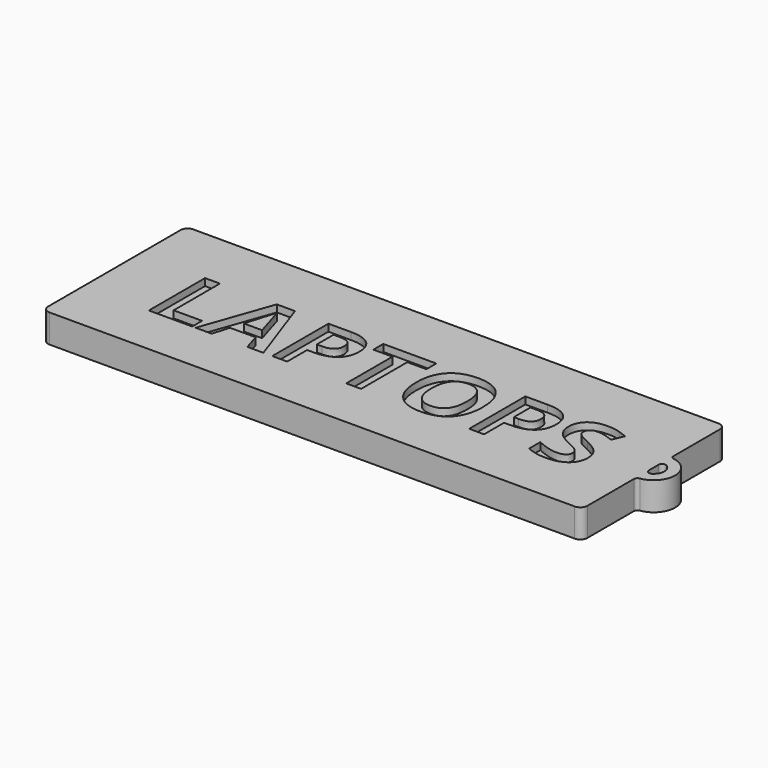
from build123d import *

# Parameters (mm, degrees)
F1_DEPTH     = 8
F2_TEXT_SIZE = 27.7777777778
F3_DEPTH     = 2


# Not quite as in the source:
# - Text() gives the source's letters only with a copy of the font that has no kerning and outlines rounded to 1/6400 em; it was checked with that copy


with BuildPart() as f1:
    # F0 (on Top) → F1 (new body)
    with BuildSketch(Plane.XY):
        with BuildLine():
            Line((-150.4, 0), (-2, 0))
            ThreePointArc((-2, 0), (-0.5857864376, 0.5857864376), (0, 2))
            Line((0, 2), (0, 18.415734535))
            ThreePointArc((0, 18.415734535), (0.2444427339, 19.0708171386), (0.8582664352, 19.4056393772))
            ThreePointArc((0.8582664352, 19.4056393772), (6.0554917678, 25.4), (0.8582664352, 31.3943606228))
            ThreePointArc((0.8582664352, 31.3943606228), (0.2444427339, 31.7291828614), (0, 32.384265465))
            Line((0, 32.384265465), (0, 48.8))
            ThreePointArc((0, 48.8), (-0.5857864376, 50.2142135624), (-2, 50.8))
            Line((-2, 50.8), (-150.4, 50.8))
            ThreePointArc((-150.4, 50.8), (-151.8142135624, 50.2142135624), (-152.4, 48.8))
            Line((-152.4, 48.8), (-152.4, 2))
            ThreePointArc((-152.4, 2), (-151.8142135624, 0.5857864376), (-150.4, 0))
        make_face()
        with BuildLine():
            ThreePointArc((1.5, 27.9980762114), (3, 25.4), (1.5, 22.8019237886))
            ThreePointArc((1.5, 22.8019237886), (0.5, 22.8019237886), (0, 23.6679491924))
            Line((0, 23.6679491924), (0, 25.4))
            Line((0, 25.4), (0, 27.1320508076))
            ThreePointArc((0, 27.1320508076), (0.5, 27.9980762114), (1.5, 27.9980762114))
        make_face(mode=Mode.SUBTRACT)
    extrude(amount=-F1_DEPTH)

    # F2 (on face) → F3 (cut)
    with BuildSketch(Plane.XY):
        with Locations((-136.3470242986, 14.4248167941)):
            Text('LAPTOPS', F2_TEXT_SIZE, font='Open Sans', font_style=FontStyle.BOLD, text_align=(TextAlign.LEFT, TextAlign.BOTTOM))
    extrude(amount=-F3_DEPTH, mode=Mode.SUBTRACT)


solid = f1.part
